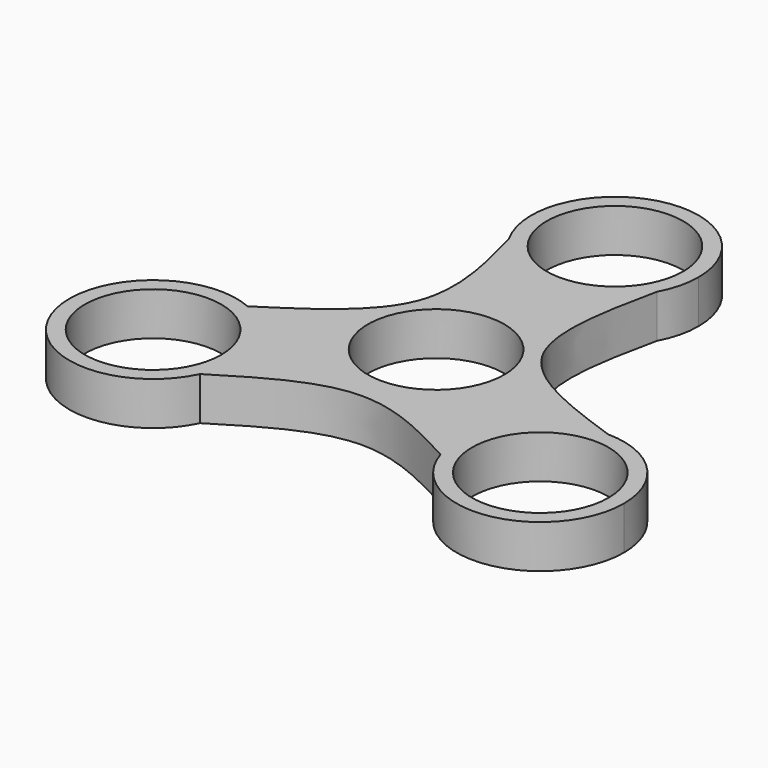
from build123d import *

# Parameters (mm, degrees)
F0_R     = 11.05
F1_DEPTH = 7


with BuildPart() as f1:
    # F0 (on Top) → F1 (new body)
    with BuildSketch(Plane.XY):
        with BuildLine():
            ThreePointArc((-12.6831392694, 4.7686977545), (-2.4234234979, -13.3315234895), (13.55, 0))
            ThreePointArc((13.55, 0), (13.1027192195, 3.4527161853), (11.7904060434, 6.6774864532))
            add(Edge.make_bspline(
                [(11.5297847403, 7.1180449452), (11.6132861066, 6.969341391), (11.7001892822, 6.8225044208), (11.7904060434, 6.6774864532)],
                knots=[0.4974758981, 0.4974758981, 0.4974758981, 0.4974758981, 0.5104096373, 0.5104096373, 0.5104096373, 0.5104096373], degree=3))
            ThreePointArc((11.5297847403, 7.1180449452), (1.1469220688, 13.5013728846), (-10.1639023184, 8.9608922359))
            add(Edge.make_bspline(
                [(-10.1639023184, 8.9608922359), (-10.7500939319, 7.4698745289), (-11.6129235501, 6.081120856), (-12.6831392694, 4.7686977545)],
                knots=[0.4943184599, 0.4943184599, 0.4943184599, 0.4943184599, 0.6210165425, 0.6210165425, 0.6210165425, 0.6210165425], degree=3))
        make_face()
        Circle(F0_R, mode=Mode.SUBTRACT)
        with BuildLine():
            ThreePointArc((11.7904060434, 6.6774864532), (13.1027192195, 3.4527161853), (13.55, 0))
            ThreePointArc((13.55, 0), (-2.4234234979, -13.3315234895), (-12.6831392694, 4.7686977545))
            add(Edge.make_bspline(
                [(-12.6831392694, 4.7686977545), (-15.884403608, 0.8429347549), (-20.9412495964, -2.399862478), (-26.0002209429, -5.6537765206)],
                knots=[0.6210165425, 0.6210165425, 0.6210165425, 0.6210165425, 1, 1, 1, 1], degree=3))
            ThreePointArc((-26.0002209429, -5.6537765206), (-20.0363711479, -10.649419061), (-17.8030151047, -18.1016717106))
            ThreePointArc((-17.8030151047, -18.1016717106), (-18.1329053392, -21.0734048392), (-19.1065129332, -23.9004374898))
            add(Edge.make_bspline(
                [(-19.1065129332, -23.9004374898), (-12.7337335325, -19.9495363252), (-0.2067317894, -12.1959048864), (12.344888234, -18.8150479155), (18.4126389706, -22.1202741428)],
                knots=[0, 0, 0, 0, 0.5079978735, 1, 1, 1, 1], degree=3))
            ThreePointArc((18.4126389706, -22.1202741428), (20.4851117611, -10.0090097929), (31.4943521465, -4.5524088583))
            add(Edge.make_bspline(
                [(11.7904060434, 6.6774864532), (15.2054475833, 1.1880144624), (23.3685436118, -1.6949988805), (31.4943521465, -4.5524088583)],
                knots=[0.5104096373, 0.5104096373, 0.5104096373, 0.5104096373, 1, 1, 1, 1], degree=3))
        make_face()
        with BuildLine():
            ThreePointArc((-10.1639023184, 8.9608922359), (1.1469220688, 13.5013728846), (11.5297847403, 7.1180449452))
            add(Edge.make_bspline(
                [(11.9294824461, 29.7776178927), (10.1390437597, 21.3188304105), (8.3180362773, 12.8376928177), (11.5297847403, 7.1180449452)],
                knots=[0, 0, 0, 0, 0.4974758981, 0.4974758981, 0.4974758981, 0.4974758981], degree=3))
            ThreePointArc((11.9294824461, 29.7776178927), (0.164433974, 22.6543411898), (-11.7700234604, 29.4899949467))
            add(Edge.make_bspline(
                [(-11.7700234604, 29.4899949467), (-9.8007963488, 22.152111828), (-7.8768484836, 14.7781671429), (-10.1639023184, 8.9608922359)],
                knots=[0, 0, 0, 0, 0.4943184599, 0.4943184599, 0.4943184599, 0.4943184599], degree=3))
        make_face()
        with BuildLine():
            ThreePointArc((44.9030151047, -18.1016717106), (40.9841525484, -8.5704760069), (31.4943521465, -4.5524088583))
            ThreePointArc((31.4943521465, -4.5524088583), (20.4851117611, -10.0090097929), (18.4126389706, -22.1202741428))
            ThreePointArc((18.4126389706, -22.1202741428), (33.3853048703, -31.4983988597), (44.9030151047, -18.1016717106))
        make_face()
        with Locations((31.3530151047, -18.1016717106)):
            Circle(F0_R, mode=Mode.SUBTRACT)
        with BuildLine():
            ThreePointArc((-17.8030151047, -18.1016717106), (-20.0363711479, -10.649419061), (-26.0002209429, -5.6537765206))
            ThreePointArc((-26.0002209429, -5.6537765206), (-44.028541405, -22.8905685576), (-19.1065129332, -23.9004374898))
            ThreePointArc((-19.1065129332, -23.9004374898), (-18.1329053392, -21.0734048392), (-17.8030151047, -18.1016717106))
        make_face()
        with Locations((-31.3530151047, -18.1016717106)):
            Circle(F0_R, mode=Mode.SUBTRACT)
        with BuildLine():
            ThreePointArc((-11.7700234604, 29.4899949467), (0.164433974, 22.6543411898), (11.9294824461, 29.7776178927))
            ThreePointArc((11.9294824461, 29.7776178927), (13.1386260154, 32.8898850425), (13.55, 36.2033434212))
            ThreePointArc((13.55, 36.2033434212), (-3.472656196, 49.3007919874), (-11.7700234604, 29.4899949467))
        make_face()
        with Locations((0, 36.2033434212)):
            Circle(F0_R, mode=Mode.SUBTRACT)
    extrude(amount=F1_DEPTH)


solid = f1.part
